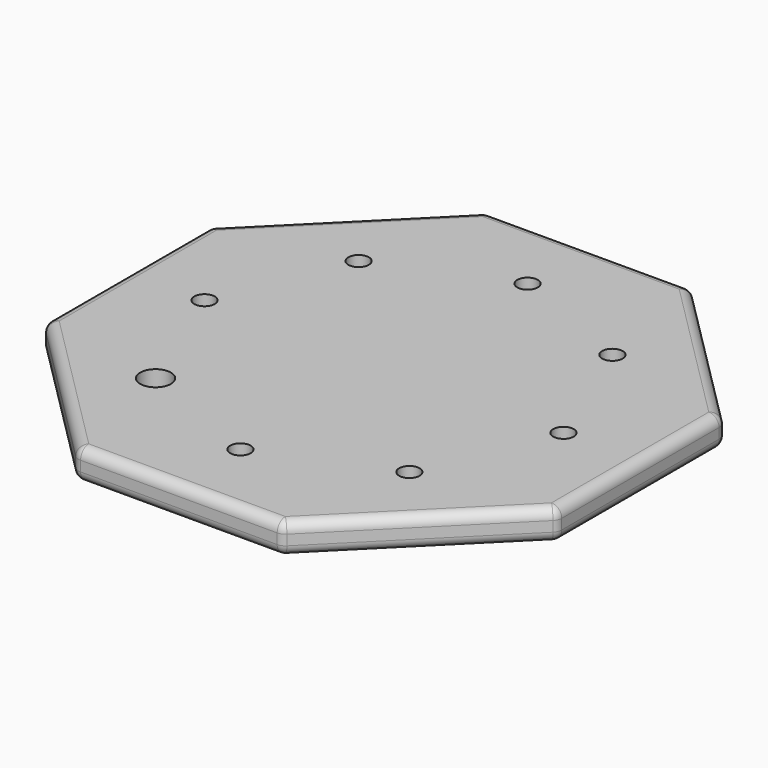
from build123d import *

# Parameters (mm, degrees)
F0_W            = 250
F0_H            = 250
F1_DEPTH        = 15
F3_R            = 5
F4_DEPTH        = 15.001
F4_COPIES_COUNT = 7
F4_COPIES_ANGLE = 270
F6_R            = 7.5
F7_DEPTH        = 15.001
F8_SIZE         = 75
F9_R            = 5


# Not quite as in the source:
# - a pattern or mirror of a feature is missing from the dataset's text; its kind, count and spacing are read off the source's solid


with BuildPart() as f1:
    # F0 (on Top) → F1 (new body)
    with BuildSketch(Plane.XY):
        Rectangle(F0_W, F0_H)
    extrude(amount=F1_DEPTH)

    # F3 (on face) → F4 (cut, through all)
    with BuildSketch(Plane.XY.offset(15)):
        with Locations((-87.5, 0)):
            Circle(F3_R)
    f4 = extrude(amount=-F4_DEPTH, mode=Mode.SUBTRACT)

    # F4_copies: F4 ×7 about axis
    f4_copies_axis = Axis((0, 0, 0), (0, 0, -1))
    for i in range(1, F4_COPIES_COUNT):
        add(f4.rotate(f4_copies_axis, i * F4_COPIES_ANGLE / (F4_COPIES_COUNT - 1)), mode=Mode.SUBTRACT)

    # F6 (on face) → F7 (cut, through all)
    with BuildSketch(Plane.XY.offset(15)):
        with Locations((-61.8718433538, -61.8718433538)):
            Circle(F6_R)
    extrude(amount=-F7_DEPTH, mode=Mode.SUBTRACT)

    # F8
    f8_edges = [f1.edges().sort_by_distance(p)[0] for p in [
        (-125, 125, 7.5),
        (-125, -125, 7.5),
        (125, -125, 7.5),
        (125, 125, 7.5),
    ]]
    chamfer(f8_edges, length=F8_SIZE)

    # F9
    f9_edges = [f1.edges().sort_by_distance(p)[0] for p in [
        (-125, 0, 15),
        (-125, 0, 0),
        (-125, 50, 7.5),
        (-125, -50, 7.5),
        (-87.5, -87.5, 0),
        (-50, -125, 7.5),
        (-87.5, -87.5, 15),
        (0, -125, 0),
        (50, -125, 7.5),
        (0, -125, 15),
        (87.5, -87.5, 0),
        (125, -50, 7.5),
        (87.5, -87.5, 15),
        (125, 0, 0),
        (125, 50, 7.5),
        (125, 0, 15),
        (87.5, 87.5, 0),
        (50, 125, 7.5),
        (87.5, 87.5, 15),
        (0, 125, 0),
        (-50, 125, 7.5),
        (0, 125, 15),
        (-87.5, 87.5, 0),
        (-87.5, 87.5, 15),
    ]]
    fillet(f9_edges, radius=F9_R)


solid = f1.part
